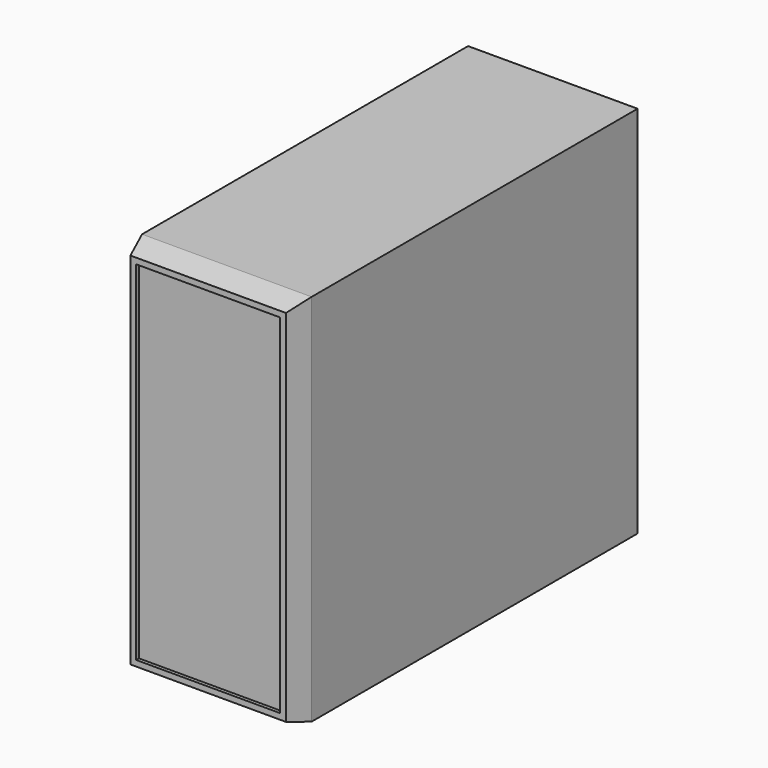
from build123d import *

# Parameters (mm, degrees)
F0_W     = 184.912
F0_H     = 407.924
F1_DEPTH = 469.9
F2_SIZE2 = 25.4
F2_SIZE  = 7.62
F3_W     = 156.972
F3_H     = 379.984
F4_DEPTH = 3.81


with BuildPart() as f1:
    # F0 (on Front) → F1 (new body)
    with BuildSketch(Plane.XZ):
        with Locations((92.456, 203.962)):
            Rectangle(F0_W, F0_H)
    extrude(amount=-F1_DEPTH)

    # F2
    f2_edges = [f1.edges().sort_by_distance(p)[0] for p in [
        (0, 0, 203.962),
        (92.456, 0, 407.924),
        (184.912, 0, 203.962),
        (92.456, 0, 0),
    ]]
    f2_side = f1.faces().sort_by_distance((92.456, 0, 203.962))[0]
    chamfer(f2_edges, length=F2_SIZE, length2=F2_SIZE2, reference=f2_side)

    # F3 (on face) → F4 (cut)
    with BuildSketch(Plane.XZ):
        with Locations((92.456, 203.962)):
            Rectangle(F3_W, F3_H)
    extrude(amount=-F4_DEPTH, mode=Mode.SUBTRACT)


solid = f1.part
